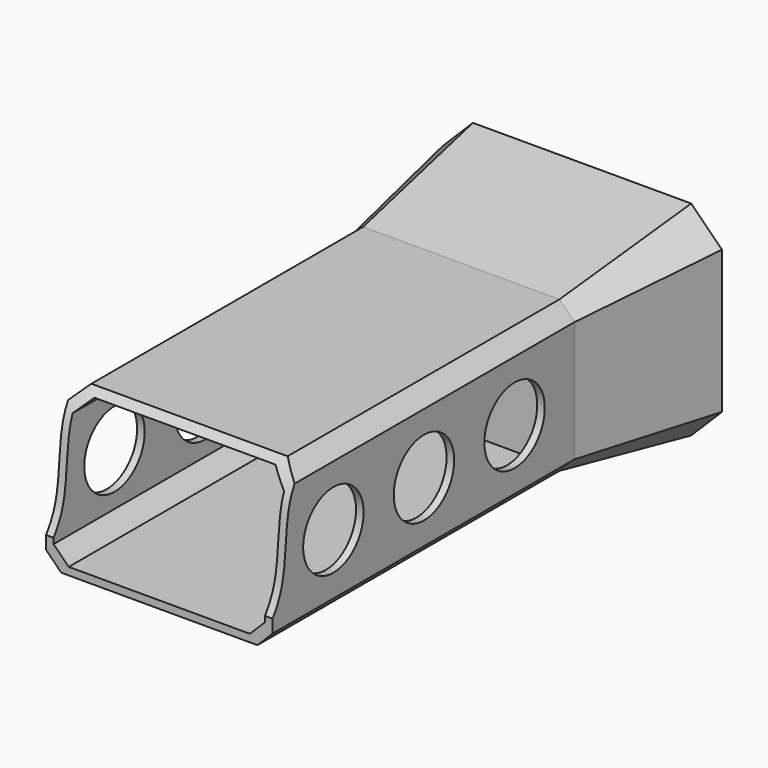
from build123d import *

# Parameters (mm, degrees)
F0_W     = 76.2
F0_H     = 50.8
F1_DEPTH = 127
F2_T     = -2.54
F3_R     = 12.7
F4_DEPTH = 76.201
F6_DEPTH = 76.201
F7_SIZE  = 5.08
F9_DEPTH = 50.8
F9_TAPER = -10
F10_T    = -2.54


with BuildPart() as f1:
    # F0 (on Front) → F1 (new body)
    with BuildSketch(Plane.XZ):
        with Locations((38.1, 25.4)):
            Rectangle(F0_W, F0_H)
    extrude(amount=F1_DEPTH)

    # F2
    f2_openings = [f1.faces().sort_by_distance(p)[0] for p in [
        (38.1, -127, 25.4),
    ]]
    offset(amount=F2_T, openings=f2_openings)

    # F3 (on face) → F4 (cut, through all)
    with BuildSketch(Plane.YZ.offset(76.2)):
        with Locations((-101.4156882687, 25.4)):
            Circle(F3_R)
        with Locations((-63.3156882687, 25.4)):
            Circle(F3_R)
        with Locations((-25.2156882687, 25.4)):
            Circle(F3_R)
    extrude(amount=-F4_DEPTH, mode=Mode.SUBTRACT)

    # F5 (on face) → F6 (cut, through all)
    with BuildSketch(Plane.YZ.offset(76.2)):
        with BuildLine():
            add(Edge.make_bspline(
                [(-114.3024048609, 50.8), (-116.3753766316, 48.2180029007), (-122.7739913645, 38.3634851462), (-120.2785073467, 21.2308461151), (-125.5979944732, 11.4326219351), (-127, 9.4929700746)],
                knots=[0.1809579396, 0.1809579396, 0.1809579396, 0.1809579396, 0.3115506916, 0.6462020469, 0.7356568333, 0.7356568333, 0.7356568333, 0.7356568333], degree=3))
            Line((-114.3024048609, 50.8), (-127, 50.8))
            Line((-127, 50.8), (-127, 9.4929700746))
        make_face()
    extrude(amount=-F6_DEPTH, mode=Mode.SUBTRACT)

    # F7
    f7_edges = [f1.edges().sort_by_distance(p)[0] for p in [
        (2.54, -64.77, 2.54),
        (73.66, -64.77, 2.54),
        (2.54, -59.366962, 48.26),
        (73.66, -59.366962, 48.26),
        (0, -57.151202, 50.8),
        (76.2, -57.151202, 50.8),
        (0, -63.5, 0),
        (76.2, -63.5, 0),
    ]]
    chamfer(f7_edges, length=F7_SIZE)

    # F8 (on face) → F9 (join)
    with BuildSketch(Plane(origin=(0, 0, 0), x_dir=(-1, 0, 0), z_dir=(0, 1, 0))):
        Polygon((0, 45.72), (-5.08, 50.8), (-71.12, 50.8), (-76.2, 45.72), (-76.2, 9.4929700837), (-76.2, 5.08), (-71.12, 0), (-5.08, 0), (0, 5.08), align=None)
    extrude(amount=F9_DEPTH, taper=F9_TAPER)

    # F10
    f10_openings = [f1.faces().sort_by_distance(p)[0] for p in [
        (38.1, 50.8, 25.4),
    ]]
    offset(amount=F10_T, openings=f10_openings, kind=Kind.INTERSECTION)


solid = f1.part
